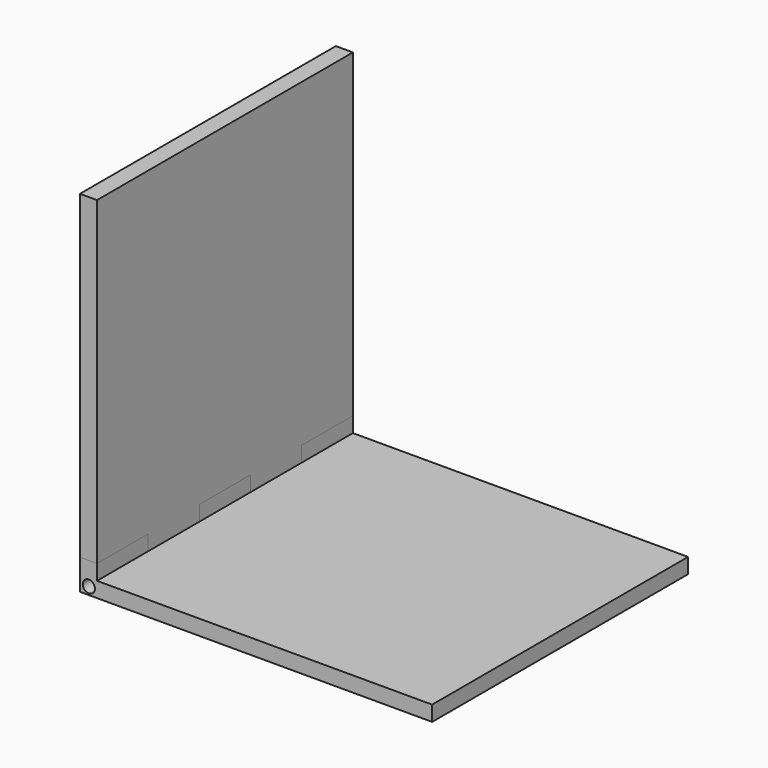
from build123d import *

# Parameters (mm, degrees)
F1_DEPTH  = 5
F3_D      = 4
F3_DEPTH  = 84.001
F4_D      = 4
F5_W      = 5.6
F5_H      = 21
F6_DEPTH  = 5
F7_W      = 21
F7_H      = 5
F8_DEPTH  = 5.6
F7_H_2    = 10
F9_W      = 5.6
F9_H      = 21
F10_DEPTH = 105


with BuildPart() as f1:
    # F0 (on Top) → F1 (new body)
    with BuildSketch(Plane.XY):
        Polygon((57.8, -52.5), (57.8, 52.5), (-57.8, 52.5), (-57.8, 31.5), (-52.2, 31.5), (-52.2, 10.5), (-57.8, 10.5), (-57.8, -10.5), (-52.2, -10.5), (-52.2, -31.5), (-57.8, -31.5), (-57.8, -52.5), align=None)
    extrude(amount=F1_DEPTH)

    # F3 (through all, one way)
    with BuildSketch(Plane(origin=(0, 31.5, 0), x_dir=(1, 0, 0), z_dir=(0, 1, 0))):
        with Locations((-54.8736937344, -2.5)):
            Circle(F3_D / 2)
    extrude(amount=-F3_DEPTH, mode=Mode.SUBTRACT)

    # F4 (through all)
    with Locations(Plane.XZ.offset(-31.5)):
        with Locations((-54.8736937344, 2.5)):
            Hole(F4_D / 2)

    # F5 (on face) → F6 (join)
    with BuildSketch(Plane.XY.offset(5)):
        with Locations((-55, 42)):
            Rectangle(F5_W, F5_H)
        with Locations((-55, 0)):
            Rectangle(F5_W, F5_H)
        with Locations((-55, -42)):
            Rectangle(F5_W, F5_H)
    extrude(amount=F6_DEPTH)


with BuildPart() as f8:
    # F7 (on face) → F8 (new body)
    with BuildSketch(Plane(origin=(-52.2, 0, 0), x_dir=(0, -1, 0), z_dir=(-1, 0, 0))):
        with Locations((-21, 7.5)):
            Rectangle(F7_W, F7_H)
        with Locations((-21, 2.5)):
            Rectangle(F7_W, F7_H)
    extrude(amount=F8_DEPTH)



with BuildPart() as f8b:
    # F7 (on face) → F8, piece 2 (new body)
    with BuildSketch(Plane(origin=(-52.2, 0, 0), x_dir=(0, -1, 0), z_dir=(-1, 0, 0))):
        with Locations((21, 5)):
            Rectangle(F7_W, F7_H_2)
    extrude(amount=F8_DEPTH)


with BuildPart() as f8_1:
    add(f8.part)

    add(f8b.part)  # F10 merges F8b
    # F9 (on face) → F10 (join)
    with BuildSketch(Plane.XY.offset(10)):
        with Locations((-55, 42)):
            Rectangle(F9_W, F9_H)
        Polygon((-57.8, 31.5), (-57.8, -31.5), (-57.8, -52.5), (-52.2, -52.5), (-52.2, 31.5), align=None)
    extrude(amount=F10_DEPTH)


solid = Compound([f1.part, f8_1.part])
